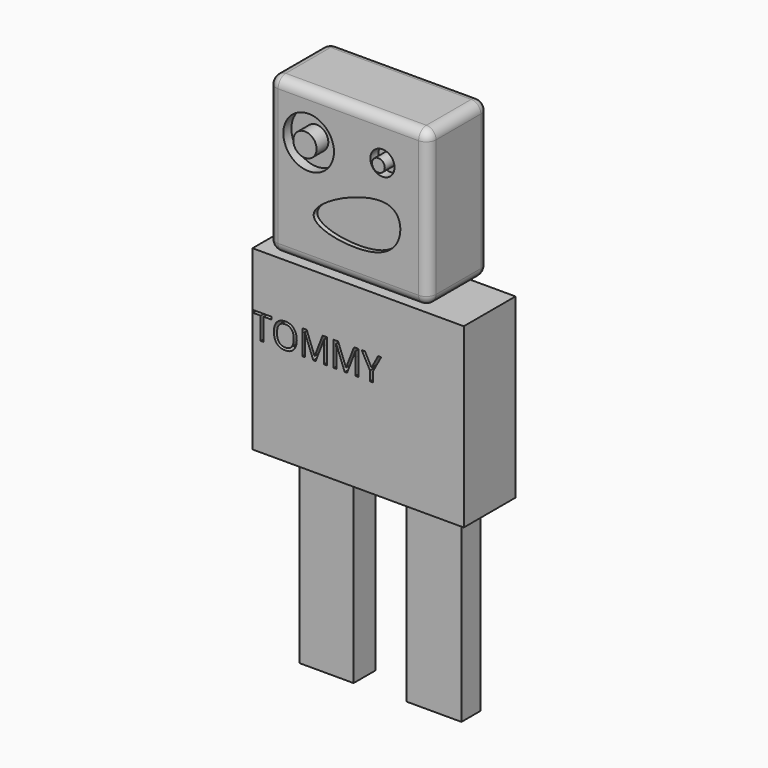
from build123d import *

# Parameters (mm, degrees)
F0_W          = 82.7635023743
F0_H          = 80.4247390479
F1_DEPTH      = 39
F2_R          = 5
F3_R          = 13.099735063
F3_R_2        = 6.2622265426
F4_DEPTH      = 5.2
F5_R          = 6.0225656801
F5_R_2        = 3.3061665955
F6_DEPTH      = 7.6
F8_DEPTH      = 2.4
F9_W          = 29.1754491627
F9_H          = 15.655121766
F10_DEPTH     = 3.8
F11_W         = 109.3486507889
F11_H         = 33.4450299852
F12_DEPTH     = 91.7
F13_W         = 27.989462018
F13_H         = 14.2319286242
F13_W_2       = 28.4638563171
F13_H_2       = 12.3343365267
F14_DEPTH     = 96.1
F15_TEXT_SIZE = 18.0137085004
F16_DEPTH     = 5


# Not quite as in the source:
# - Text() gives the source's letters only with a copy of the font that has no kerning and outlines rounded to 1/6400 em; it was checked with that copy


with BuildPart() as f1:
    # F0 (on Front) → F1 (new body)
    with BuildSketch(Plane.XZ):
        with Locations((-59.0552119538, 16.1438444629)):
            Rectangle(F0_W, F0_H)
    extrude(amount=F1_DEPTH)

    # F2
    f2_edges = [f1.edges().sort_by_distance(p)[0] for p in [
        (-59.055212, -39, 56.356214),
        (-100.436963, -39, 16.143844),
        (-100.436963, -19.5, 56.356214),
        (-100.436963, -19.5, -24.068525),
        (-59.055212, -39, -24.068525),
        (-17.673461, -39, 16.143844),
        (-17.673461, -19.5, -24.068525),
        (-17.673461, -19.5, 56.356214),
        (-17.673461, 0, 16.143844),
        (-59.055212, 0, 56.356214),
        (-59.055212, 0, -24.068525),
        (-100.436963, 0, 16.143844),
    ]]
    fillet(f2_edges, radius=F2_R)

    # F3 (on face) → F4 (cut)
    with BuildSketch(Plane.XZ.offset(39)):
        with Locations((-79.6085447073, 32.0218391716)):
            Circle(F3_R)
        with Locations((-41.4195358753, 35.1054221392)):
            Circle(F3_R_2)
    extrude(amount=-F4_DEPTH, mode=Mode.SUBTRACT)

    # F5 (on face) → F6 (join)
    with BuildSketch(Plane.XZ.offset(33.8)):
        with Locations((-79.6085447073, 32.0218391716)):
            Circle(F5_R)
        with Locations((-41.596326977, 34.9469408393)):
            Circle(F5_R_2)
    extrude(amount=F6_DEPTH)

    # F7 (on face) → F8 (cut)
    with BuildSketch(Plane.XZ.offset(39)):
        with BuildLine():
            add(Edge.make_bspline(
                [(-76.9993588328, 0), (-76.6186190977, 7.3803416775), (-36.015145433, 26.1951862037), (-29.4571348745, 3.3810787814), (-44.3112752898, -11.8288400701), (-77.3264890159, -6.3411624826), (-76.9993588328, 0)],
                knots=[0, 0, 0, 0, 0.3185643971, 0.5055981768, 0.7262906391, 1, 1, 1, 1], degree=3))
        make_face()
    extrude(amount=-F8_DEPTH, mode=Mode.SUBTRACT)

    # F9 (on face) → F10 (join)
    with BuildSketch(Plane(origin=(0, 0, -24.068525061), x_dir=(1, 0, 0), z_dir=(0, 0, -1))):
        with Locations((-57.193255052, 20.1618992724)):
            Rectangle(F9_W, F9_H)
    extrude(amount=F10_DEPTH)

    # F11 (on face) → F12 (join)
    with BuildSketch(Plane(origin=(0, 0, -27.868525061), x_dir=(1, 0, 0), z_dir=(0, 0, -1))):
        with Locations((-56.7188580753, 18.8573042396)):
            Rectangle(F11_W, F11_H)
    extrude(amount=F12_DEPTH)

    # F13 (on face) → F14 (join)
    with BuildSketch(Plane(origin=(0, 0, -119.568525061), x_dir=(1, 0, 0), z_dir=(0, 0, -1))):
        with Locations((-81.0542702675, 18.5015066527)):
            Rectangle(F13_W, F13_H)
        with Locations((-26.0241511278, 18.7387051992)):
            Rectangle(F13_W_2, F13_H_2)
    extrude(amount=F14_DEPTH)

    # F15 (on face) → F16 (cut)
    with BuildSketch(Plane.XZ.offset(35.5798192322)):
        with Locations((-111.3931834698, -68.7506571412)):
            Text('TOMMY', F15_TEXT_SIZE, font='Open Sans', text_align=(TextAlign.LEFT, TextAlign.BOTTOM))
    extrude(amount=-F16_DEPTH, mode=Mode.SUBTRACT)


solid = f1.part
